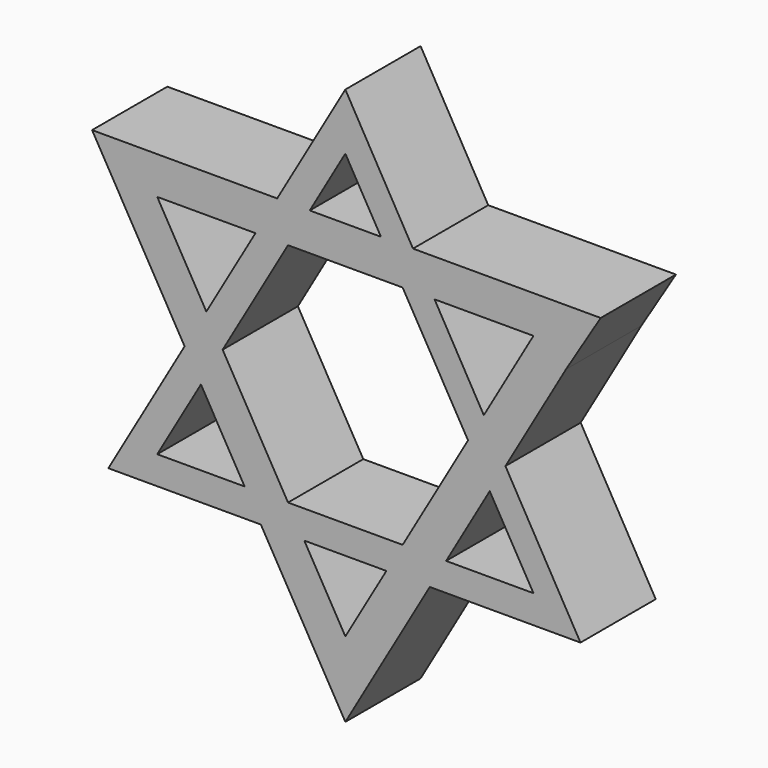
from build123d import *

# Parameters (mm, degrees)
F1_DEPTH = 10


with BuildPart() as f1:
    # F0 (on Front) → F1 (new body)
    with BuildSketch(Plane.XZ):
        Polygon((-10.7119849175, -24.0873143706), (-6.0931825641, -24.0873143706), (-13.046591282, -12.0436571853), (-15.3559924588, -16.0436573585), align=None)
        Polygon((4.3611317565, -27.0873143706), (0, -34.6410161514), (-4.3611317565, -27.0873143706), (-8.9799341099, -27.0873143706), (0, -42.6410164977), (8.9799341099, -27.0873143706), align=None)
        Polygon((13.046591282, -12.0436571853), (6.0931825641, -24.0873143706), (10.7119849175, -24.0873143706), (15.3559924588, -16.0436573585), align=None)
        Polygon((20, 0), (14.7208913197, -9.143684453), (17.0212680072, -13.1593155), (23.4641017651, -2.0000000866), (27.1496195346, 4.00000019), (20, 4.00000019), (7.1914581155, 4.00000019), (9.4828805792, 0), align=None)
        Polygon((-3.7837813776, 4.00000019), (-6.0931825641, 0), (6.0931825641, 0), (3.7837813776, 4.00000019), align=None)
        Polygon((-17.0880432663, -13.0436573585), (-14.7786420896, -9.0436571853), (-20, 0), (-9.5572841792, 0), (-7.2478829927, 4.00000019), (-20, 4.00000019), (-26.9282035399, 4.00000019), (-23.4641017651, -2.0000000866), align=None)
        Polygon((-15.3559924588, -16.0436573585), (-13.046591282, -12.0436571853), (-14.7786420896, -9.0436571853), (-17.0880432663, -13.0436573585), align=None)
        Polygon((-8.9799341099, -27.0873143706), (-4.3611317565, -27.0873143706), (-6.0931825641, -24.0873143706), (-10.7119849175, -24.0873143706), align=None)
        Polygon((6.0931825641, -24.0873143706), (4.3611317565, -27.0873143706), (8.9799341099, -27.0873143706), (10.7119849175, -24.0873143706), align=None)
        Polygon((14.7208913197, -9.143684453), (13.046591282, -12.0436571853), (15.3559924588, -16.0436573585), (17.0212680072, -13.1593155), align=None)
        Polygon((3.7837813776, 4.00000019), (6.0931825641, 0), (9.4828805792, 0), (7.1914581155, 4.00000019), align=None)
        Polygon((-9.5572841792, 0), (-6.0931825641, 0), (-3.7837813776, 4.00000019), (-7.2478829927, 4.00000019), align=None)
        Polygon((-14.7786420896, -9.0436571853), (-13.046591282, -12.0436571853), (-6.0931825641, 0), (-9.5572841792, 0), align=None)
        Polygon((-25.1961524227, -27.0873143706), (-8.9799341099, -27.0873143706), (-10.7119849175, -24.0873143706), (-20, -24.0873143706), (-15.3559924588, -16.0436573585), (-17.0880432663, -13.0436573585), align=None)
        Polygon((-6.0931825641, -24.0873143706), (-4.3611317565, -27.0873143706), (4.3611317565, -27.0873143706), (6.0931825641, -24.0873143706), align=None)
        Polygon((10.7119849175, -24.0873143706), (8.9799341099, -27.0873143706), (25, -27.0873143706), (17.0212680072, -13.1593155), (15.3559924588, -16.0436573585), (20, -24.0873143706), align=None)
        Polygon((6.0931825641, 0), (13.046591282, -12.0436571853), (14.7208913197, -9.143684453), (9.4828805792, 0), align=None)
        Polygon((-7.2478829927, 4.00000019), (-3.7837813776, 4.00000019), (0, 10.5537017807), (3.7837813776, 4.00000019), (7.1914581155, 4.00000019), (0, 16.5537017807), align=None)
    extrude(amount=F1_DEPTH)


solid = f1.part
